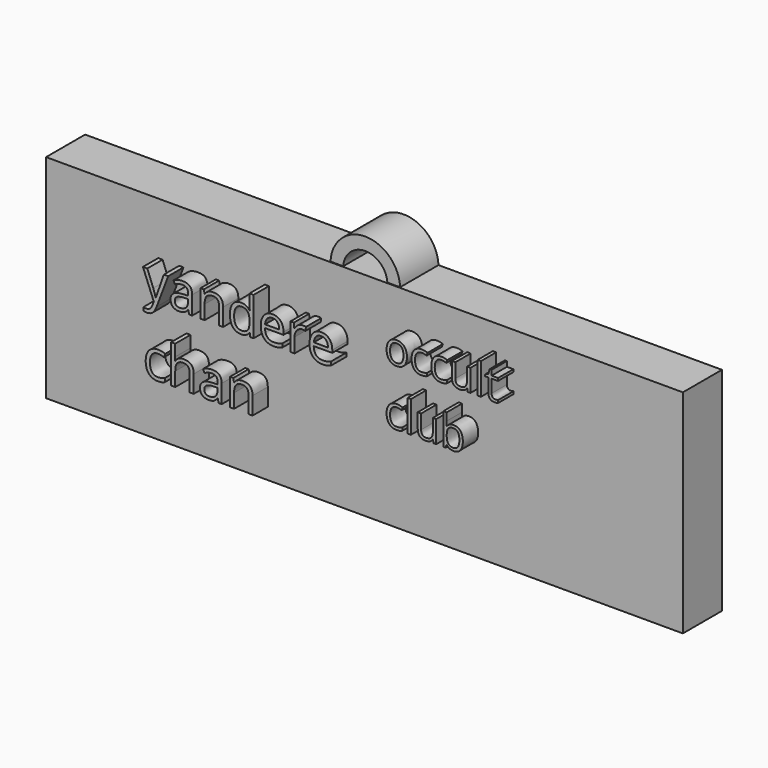
from build123d import *

# Parameters (mm, degrees)
F0_W         = 76.2
F0_H         = 25.4
F1_DEPTH     = 5.842
F2_TEXT_SIZE = 6.0196642557
F3_DEPTH     = 2.286
F4_TEXT_SIZE = 4.9476253076
F5_DEPTH     = 8.128
F7_DEPTH     = 5.7404


# Not quite as in the source:
# - Text() gives the source's letters only with a copy of the font that has no kerning and outlines rounded to 1/6400 em; it was checked with that copy


with BuildPart() as f1:
    # F0 (on Front) → F1 (new body)
    with BuildSketch(Plane.XZ):
        with Locations((5.4863984644, 8.8899998598)):
            Rectangle(F0_W, F0_H)
    extrude(amount=F1_DEPTH)

    # F2 (on face) → F3 (join)
    with BuildSketch(Plane.XZ.offset(5.842)):
        with Locations((-19.1995371133, 12.0984399691)):
            Text('yandere', F2_TEXT_SIZE, font='Open Sans', text_align=(TextAlign.LEFT, TextAlign.BOTTOM))
        with Locations((-19.1995371133, 3.9116965814)):
            Text('chan', F2_TEXT_SIZE, font='Open Sans', text_align=(TextAlign.LEFT, TextAlign.BOTTOM))
    extrude(amount=F3_DEPTH)

    # F4 (on Front) → F5 (join)
    with BuildSketch(Plane.XZ):
        with Locations((9.6858823672, 14.78151232)):
            Text('occult', F4_TEXT_SIZE, font='Open Sans', text_align=(TextAlign.LEFT, TextAlign.BOTTOM))
        with Locations((9.6858823672, 8.0527419017)):
            Text('club', F4_TEXT_SIZE, font='Open Sans', text_align=(TextAlign.LEFT, TextAlign.BOTTOM))
    extrude(amount=F5_DEPTH)

    # F6 (on Front) → F7 (join)
    with BuildSketch(Plane.XZ):
        with BuildLine():
            Line((8.1458926029, 21.5480966251), (9.6702348404, 21.5741782203))
            ThreePointArc((9.6702348404, 21.5741782203), (5.4977204304, 25.5817346864), (1.3375751986, 21.561339559))
            Line((1.3375751986, 21.561339559), (2.8640232398, 21.5767649973))
            ThreePointArc((2.8640232398, 21.5767649973), (5.5185014792, 24.0576999184), (8.1458926029, 21.5480966251))
        make_face()
    extrude(amount=F7_DEPTH)


solid = f1.part
